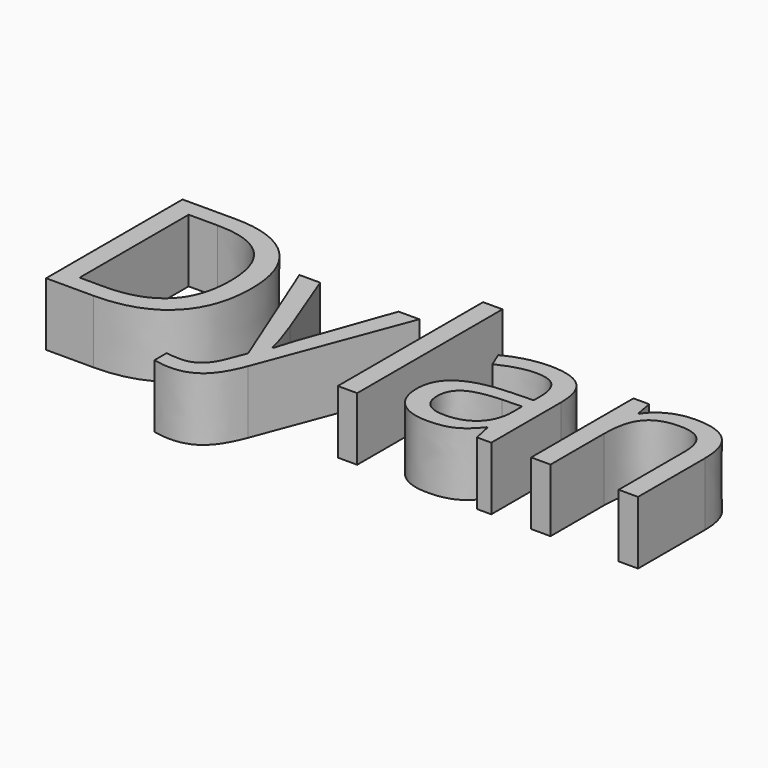
from build123d import *

# Parameters (mm, degrees)
F0_TEXT_SIZE = 96.2064271764
F1_DEPTH     = 25.4


# Not quite as in the source:
# - Text() gives the source's letters only with a copy of the font that has no kerning and outlines rounded to 1/6400 em; it was checked with that copy


with BuildPart() as f1:
    # F0 (on Top) → F1 (new body)
    with BuildSketch(Plane.XY):
        with Locations((-665.709459296, -56.5201670192)):
            Text('Dylan', F0_TEXT_SIZE, font='Open Sans', text_align=(TextAlign.LEFT, TextAlign.BOTTOM))
    extrude(amount=F1_DEPTH)


solid = f1.part
